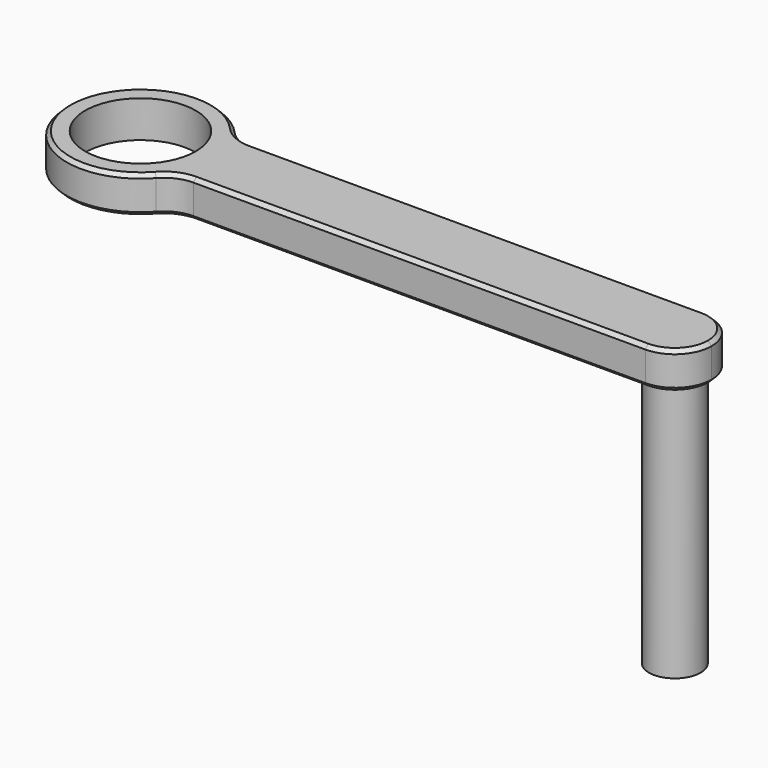
from build123d import *

# Parameters (mm, degrees)
F0_R     = 7
F1_DEPTH = 10
F2_DEPTH = 10.001
F3_R     = 9.99999
F4_SIZE  = 1
F5_R     = 7
F6_DEPTH = 80


# Not quite as in the source:
# - a fillet or chamfer is up to 0.001 mm smaller than in the source, because OpenCascade refuses the exact size


with BuildPart() as f1:
    # F0 (on Top) → F1 (new body)
    with BuildSketch(Plane.XY):
        with BuildLine():
            Line((0, -20), (0, 0))
            Line((0, 0), (-137.6794919243, 0))
            ThreePointArc((-137.6794919243, 0), (-135.6814834742, -4.8236190979), (-135, -10))
            ThreePointArc((-135, -10), (-135.6814834742, -15.1763809021), (-137.6794919243, -20))
            Line((-137.6794919243, -20), (0, -20))
        make_face()
        with Locations((-10, -10)):
            Circle(F0_R, mode=Mode.SUBTRACT)
        with BuildLine():
            Line((-143.8196601125, 0), (-137.6794919243, 0))
            ThreePointArc((-137.6794919243, 0), (-175, -10), (-137.6794919243, -20))
            Line((-137.6794919243, -20), (-143.8196601125, -20))
            ThreePointArc((-143.8196601125, -20), (-170, -10), (-143.8196601125, 0))
        make_face()
        with BuildLine():
            ThreePointArc((-135, -10), (-135.6814834742, -4.8236190979), (-137.6794919243, 0))
            Line((-137.6794919243, 0), (-143.8196601125, 0))
            ThreePointArc((-143.8196601125, 0), (-140.9874146156, -4.6476686534), (-140, -10))
            ThreePointArc((-140, -10), (-140.9874146156, -15.3523313466), (-143.8196601125, -20))
            Line((-143.8196601125, -20), (-137.6794919243, -20))
            ThreePointArc((-137.6794919243, -20), (-135.6814834742, -15.1763809021), (-135, -10))
        make_face()
    extrude(amount=F1_DEPTH)

    # F0 (on Top) → F2 (cut, through all)
    with BuildSketch(Plane.XY):
        with BuildLine():
            Line((-165, 0), (-143.8196601125, 0))
            ThreePointArc((-143.8196601125, 0), (-170, -10), (-143.8196601125, -20))
            Line((-143.8196601125, -20), (-165, -20))
            Line((-165, -20), (-165, 0))
        make_face()
        with BuildLine():
            ThreePointArc((-140, -10), (-140.9874146156, -4.6476686534), (-143.8196601125, 0))
            Line((-143.8196601125, 0), (-165, 0))
            Line((-165, 0), (-165, -20))
            Line((-165, -20), (-143.8196601125, -20))
            ThreePointArc((-143.8196601125, -20), (-140.9874146156, -15.3523313466), (-140, -10))
        make_face()
        with Locations((-10, -10)):
            Circle(F0_R)
    extrude(amount=F2_DEPTH, mode=Mode.SUBTRACT)

    # F3 (radius 10 in the source; OpenCascade refuses exactly that, so slightly less here)
    f3_edges = [f1.edges().sort_by_distance(p)[0] for p in [
        (0, -20, 5),
        (0, 0, 5),
        (-137.679492, -20, 5),
        (-137.679492, 0, 5),
    ]]
    fillet(f3_edges, radius=F3_R)

    # F4
    f4_edges = [f1.edges().sort_by_distance(p)[0] for p in [
        (-71.319657, -20, 0),
        (-2.928929, -2.928929, 10),
        (-71.319657, -20, 10),
        (-136.721804, -20.87129, 0),
        (-2.928929, -17.071071, 0),
        (-175, -10, 0),
        (0, -10, 0),
        (-136.721804, 0.87129, 0),
        (-2.928929, -2.928929, 0),
        (-71.319657, 0, 0),
        (-136.721804, -20.87129, 10),
        (-2.928929, -17.071071, 10),
        (-175, -10, 10),
        (0, -10, 10),
        (-136.721804, 0.87129, 10),
        (-71.319657, 0, 10),
    ]]
    chamfer(f4_edges, length=F4_SIZE)

    # F5 (on face) → F6 (join)
    with BuildSketch(Plane.XY.offset(10)):
        with Locations((-10, -10)):
            Circle(F5_R)
    extrude(amount=-F6_DEPTH)


solid = f1.part
